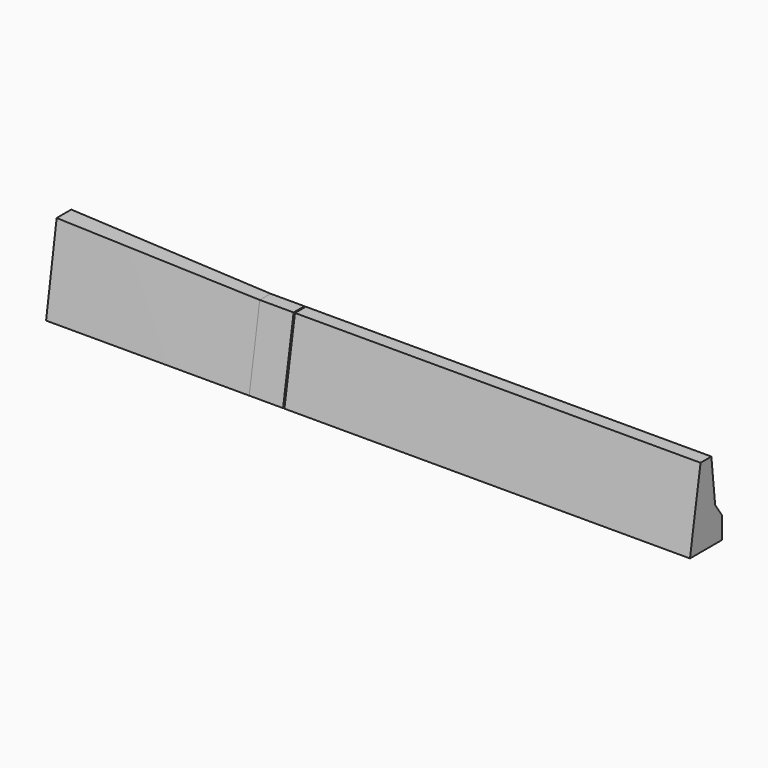
from build123d import *

# Parameters (mm, degrees)
F11_DEPTH = 5990


with BuildPart() as f6:
    # F5 (on offset) → F6 section 0
    with BuildSketch(Plane.YZ.offset(3780)):
        Polygon((-125, 0), (465, 0), (465, 325), (340, 505), (270, 1165), (70, 1165), align=None)
    # F4 (on offset) → F6 section 1
    with BuildSketch(Plane.YZ.offset(4280)):
        Polygon((-125, 0), (465, 0), (465, 325), (340, 505), (270, 1165), (70, 1165), align=None)
    loft()


with BuildPart() as f8:
    # F7 (on offset) → F8 section 0
    with BuildSketch(Plane.YZ.offset(780)):
        Polygon((-125, 0), (465, 0), (465, 325), (340, 505), (340, 1255.1641464233), (70, 1255.1641464233), align=None)
    # F5 (on offset) → F8 section 1
    with BuildSketch(Plane.YZ.offset(3780)):
        Polygon((-125, 0), (465, 0), (465, 325), (340, 505), (270, 1165), (70, 1165), align=None)
    loft()


with BuildPart() as f11:
    # F10 (on offset) → F11 (new body)
    with BuildSketch(Plane.YZ.offset(4300)):
        Polygon((-125, 0), (465, 0), (465, 325), (340, 505), (270, 1165), (70, 1165), align=None)
    extrude(amount=F11_DEPTH)


solid = Compound([f6.part, f8.part, f11.part])
